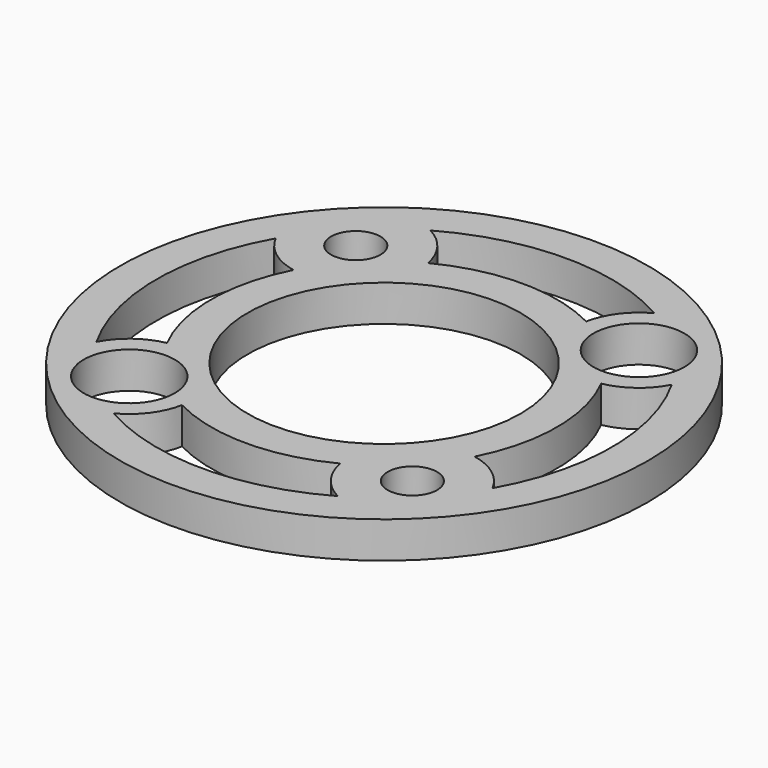
from build123d import *

# Parameters (mm, degrees)
F0_R            = 23.01875
F0_R_2          = 3.96875
F0_R_3          = 2.15265
F0_R_4          = 11.90625
F1_DEPTH        = 3.175
F3_DEPTH        = 3.175
F3_COPIES_COUNT = 4


# Not quite as in the source:
# - a pattern or mirror of a feature is missing from the dataset's text; its kind, count and spacing are read off the source's solid


with BuildPart() as f1:
    # F0 (on Top) → F1 (new body)
    with BuildSketch(Plane.XY):
        Circle(F0_R)
        with Locations((-12.3478521665, -12.3478521665)):
            Circle(F0_R_2, mode=Mode.SUBTRACT)
        with Locations((12.3478521665, -12.3478521665)):
            Circle(F0_R_3, mode=Mode.SUBTRACT)
        with Locations((-12.3478521665, 12.3478521665)):
            Circle(F0_R_3, mode=Mode.SUBTRACT)
        Circle(F0_R_4, mode=Mode.SUBTRACT)
        with Locations((12.3478521665, 12.3478521665)):
            Circle(F0_R_2, mode=Mode.SUBTRACT)
    extrude(amount=F1_DEPTH)

    # F2 (on face) → F3 (cut, through all)
    with BuildSketch(Plane.XY.offset(3.175)):
        with BuildLine():
            ThreePointArc((-6.8946489019, 13.4129757356), (0, 15.08125), (6.8946489019, 13.4129757356))
            ThreePointArc((6.8946489019, 13.4129757356), (7.8938999882, 15.6696324205), (9.7719120136, 17.2709047146))
            ThreePointArc((9.7719120136, 17.2709047146), (0, 19.84375), (-9.7719120136, 17.2709047146))
            ThreePointArc((-9.7719120136, 17.2709047146), (-7.8938999882, 15.6696324205), (-6.8946489019, 13.4129757356))
        make_face()
    f3 = extrude(amount=-F3_DEPTH, mode=Mode.SUBTRACT)

    # F3_copies: F3 ×4 about axis
    f3_copies_axis = Axis((0, 0, 0), (0, 0, 1))
    for i in range(1, F3_COPIES_COUNT):
        add(f3.rotate(f3_copies_axis, i * 360 / F3_COPIES_COUNT), mode=Mode.SUBTRACT)


solid = f1.part
